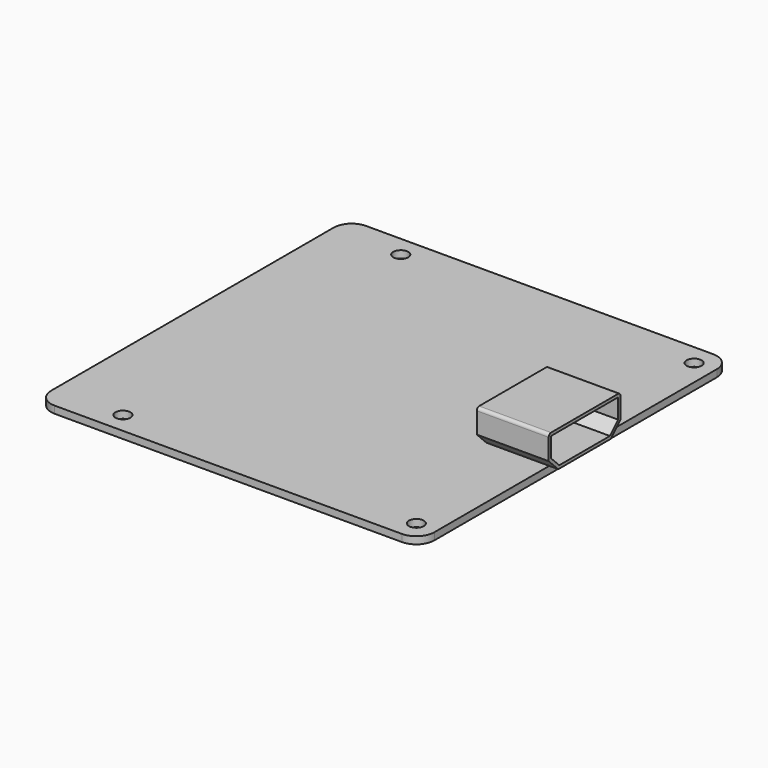
from build123d import *

# Parameters (mm, degrees)
F0_W     = 64
F0_H     = 65
F0_R     = 1.25
F1_DEPTH = 1.2
F2_R     = 3
F3_W     = 12
F3_H     = 15
F4_DEPTH = 6
F5_SIZE  = 2
F6_R     = 0.5
F7_T     = 0.5


# Not quite as in the source:
# - a shell that OpenCascade refuses in one call is made with other operations: the cavity is built on its own and cut out


with BuildPart() as f1:
    # F0 (on Top) → F1 (new body)
    with BuildSketch(Plane.XY):
        Rectangle(F0_W, F0_H)
        with Locations((-20.4, -29)):
            Circle(F0_R, mode=Mode.SUBTRACT)
        with Locations((28.6, -29)):
            Circle(F0_R, mode=Mode.SUBTRACT)
        with Locations((-20.4, 29)):
            Circle(F0_R, mode=Mode.SUBTRACT)
        with Locations((28.6, 29)):
            Circle(F0_R, mode=Mode.SUBTRACT)
    extrude(amount=F1_DEPTH)

    # F2
    f2_edges = [f1.edges().sort_by_distance(p)[0] for p in [
        (-32, 32.5, 0.6),
        (32, 32.5, 0.6),
        (32, -32.5, 0.6),
        (-32, -32.5, 0.6),
    ]]
    fillet(f2_edges, radius=F2_R)


with BuildPart() as f4:
    # F3 (on face) → F4 (new body)
    with BuildSketch(Plane.XY.offset(1.2)):
        with Locations((27.5, 0)):
            Rectangle(F3_W, F3_H)
    extrude(amount=F4_DEPTH)

    # F5
    f5_edges = [f4.edges().sort_by_distance(p)[0] for p in [
        (27.5, -7.5, 1.2),
        (27.5, 7.5, 1.2),
    ]]
    chamfer(f5_edges, length=F5_SIZE)

    # F6
    f6_edges = [f4.edges().sort_by_distance(p)[0] for p in [
        (27.5, -7.5, 7.2),
        (27.5, 7.5, 7.2),
    ]]
    fillet(f6_edges, radius=F6_R)

    # F7: shell of thickness 0.5, made by hand


with BuildPart() as f7_core1:
    # F7_t2: copy of F4
    add(f4.part)

    # the walls: a layer under each face that stays
    f7_faces = [f7_core1.faces().sort_by_distance(p)[0] for p in [
        (27.5, -7.5, 4.95),
        (27.5, -6.5, 2.2),
        (27.5, 0, 7.2),
        (27.5, 0, 1.2),
        (27.5, 6.5, 2.2),
        (27.5, 7.5, 4.95),
        (21.5, 0, 4.2),
    ]]
    thicken(f7_faces, amount=-F7_T, mode=Mode.SUBTRACT)


with BuildPart() as f4_1:
    add(f4.part)

    # what is left inside the walls is the cavity
    f7_cavity = [f7_core1.part.solids().sort_by_distance(p)[0] for p in [
        (27.75, -2.333333, 6.695),
    ]]
    add(f7_cavity, mode=Mode.SUBTRACT)


solid = Compound([f1.part, f4_1.part])
